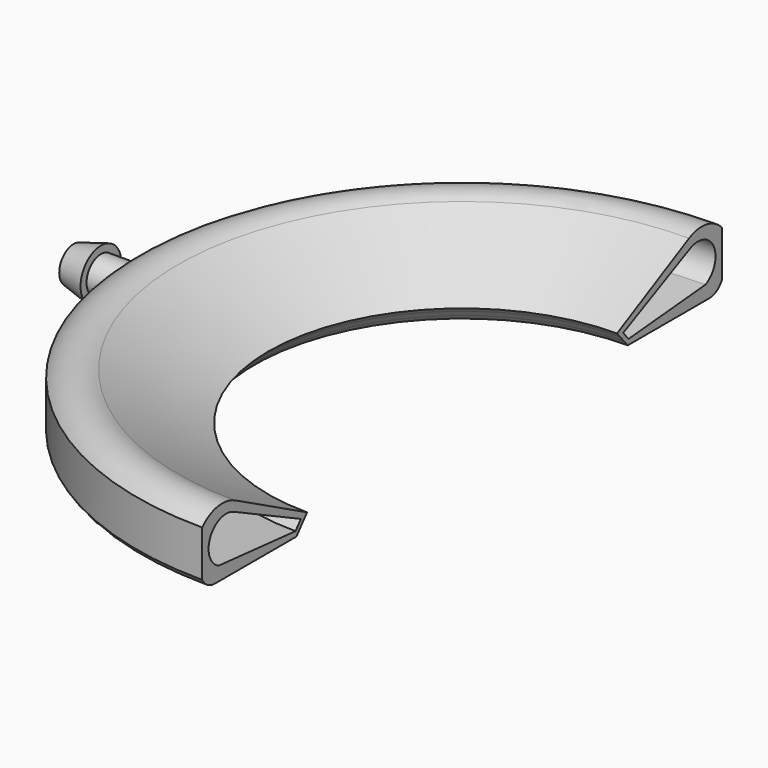
from build123d import *

# Parameters (mm, degrees)
F4_W     = 51.4225922525
F4_H     = 7.856229553
F5_DEPTH = 26


# Not quite as in the source:
# - a feature names something its author has since deleted; it is built from what else it names


with BuildPart() as f1:
    # F0 (on Front) → F1 (revolve)
    with BuildSketch(Plane.XZ):
        with BuildLine():
            Line((22.3186584817, 4.9634656969), (15.2303930372, 1.2544910423))
            Line((15.2303930372, 1.2544910423), (15.488850391, 0.9470738952))
            Line((15.488850391, 0.9470738952), (15.5328564546, 0.894731726))
            Line((15.5328564546, 0.894731726), (15.8405525238, 1.0429841968))
            Line((15.8405525238, 1.0429841968), (22.4313864066, 4.2185444515))
            ThreePointArc((22.4313864066, 4.2185444515), (24.744105662, 3.4097946744), (23.9353558848, 1.097075419))
            Line((23.9353558848, 1.097075419), (16.3696151821, 0.4137007552))
            Line((16.3696151821, 0.4137007552), (15.9677918852, 0.3774061119))
            Line((15.9677918852, 0.3774061119), (16.2850916386, 0))
            Line((16.2850916386, 0), (24.2850916386, 0))
            ThreePointArc((24.2850916386, 0), (25.023915829, 0.2087553322), (25.5442474517, 0.7732860891))
            Line((25.5442474517, 0.7732860891), (25.5442474517, 4.3952541752))
            ThreePointArc((25.5442474517, 4.3952541752), (24.028202675, 5.2285828576), (22.3186584817, 4.9634656969))
        make_face()
        Polygon((15.8405525238, 1.0429841968), (15.5328564546, 0.894731726), (15.9677918852, 0.3774061119), (16.3696151821, 0.4137007552), align=None)
    revolve(axis=Axis((0, 0, 1.8443568842), (0, 0, 1)))

    # F2 (on Front) → F3 (revolve)
    with BuildSketch(Plane.XZ):
        Polygon((-25.3970567137, 3.7070766557), (-28.3970567137, 3.7070766557), (-28.3970567137, 4.2962685693), (-30.5454257131, 3.7070766557), (-30.5454257131, 3.2924627885), (-25.5454257131, 3.2924627885), align=None)
    revolve(axis=Axis((-26.2971473858, 0, 2.2924627885), (-1, 0, 0)))

    # F4 (on Right) → F5 (cut)
    with BuildSketch(Plane.YZ):
        with Locations((-0.0007599592, 2.6581416605)):
            Rectangle(F4_W, F4_H)
    extrude(amount=F5_DEPTH, mode=Mode.SUBTRACT)


solid = f1.part
